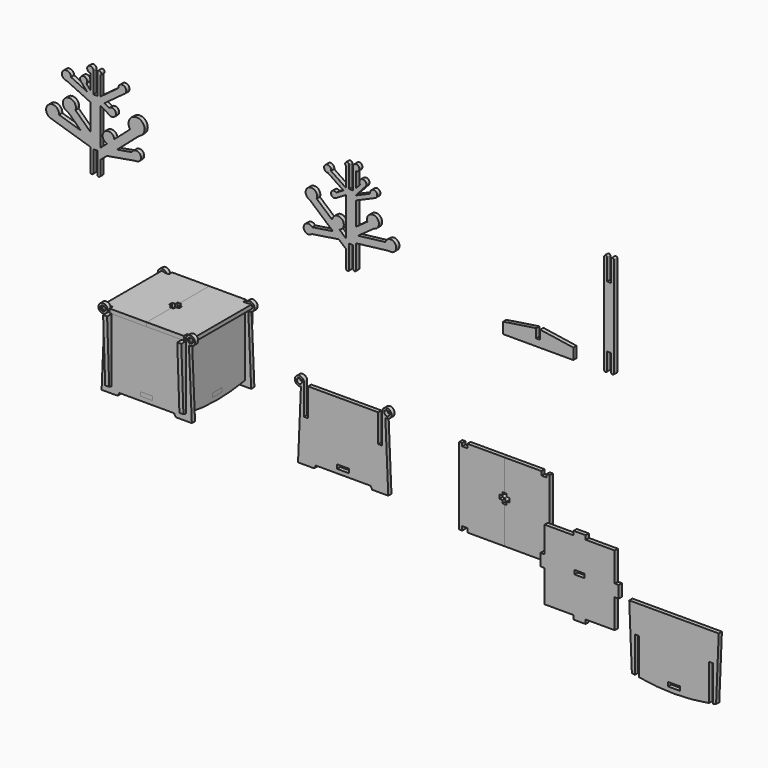
from build123d import *

# Parameters (mm, degrees)
F0_W      = 20
F0_H      = 60
F0_W_2    = 60
F0_H_2    = 20
F1_DEPTH  = 20
F2_W      = 145
F2_H      = 20
F3_DEPTH  = 20
F6_W      = 20
F6_H      = 140
F7_DEPTH  = 20
F9_W      = 15
F9_H      = 20
F9_H_2    = 15
F9_W_2    = 175
F9_W_3    = 185
F9_W_4    = 10
F10_DEPTH = 20
F13_DEPTH = 20
F18_DEPTH = 20
F19_W     = 15
F19_H     = 20
F19_W_2   = 20
F20_DEPTH = 335
F19_H_2   = 15
F21_DEPTH = 335
F23_ANGLE = 90
F27_ANGLE = -90


# Not quite as in the source:
# - a feature names something its author has since deleted; it is built from what else it names


with BuildPart() as f1:
    # F0 (on Top) → F1 (new body)
    with BuildSketch(Plane.XY):
        Polygon((394.9682962894, 292.9871472716), (249.9682962894, 292.9871472716), (249.9682962894, 133.2951399684), (269.9682962894, 133.2951399684), (269.9682962894, 73.2951399684), (249.9682962894, 73.2951399684), (249.9682962894, -57.0128527284), (394.9682962894, -57.0128527284), (394.9682962894, -37.0128527284), (454.9682962894, -37.0128527284), (454.9682962894, -57.0128527284), (599.9682962894, -57.0128527284), (599.9682962894, 87.9871472716), (579.9682962894, 87.9871472716), (579.9682962894, 147.9871472716), (599.9682962894, 147.9871472716), (599.9682962894, 292.9871472716), (454.9682962894, 292.9871472716), (454.9682962894, 272.9871472716), (394.9682962894, 272.9871472716), align=None)
        with Locations((239.9682962894, 103.2951399684)):
            Rectangle(F0_W, F0_H)
        with Locations((424.9682962894, 302.9871472716)):
            Rectangle(F0_W_2, F0_H_2)
        with Locations((609.9682962894, 117.9871472716)):
            Rectangle(F0_W, F0_H)
        with Locations((424.9682962894, -67.0128527284)):
            Rectangle(F0_W_2, F0_H_2)
        with Locations((424.9682962894, -47.0128527284)):
            Rectangle(F0_W_2, F0_H_2)
        with Locations((589.9682962894, 117.9871472716)):
            Rectangle(F0_W, F0_H)
        with Locations((424.9682962894, 282.9871472716)):
            Rectangle(F0_W_2, F0_H_2)
        with Locations((259.9682962894, 103.2951399684)):
            Rectangle(F0_W, F0_H)
    extrude(amount=F1_DEPTH)


with BuildPart() as f3:
    # F2 (on face) → F3 (new body)
    with BuildSketch(Plane.XZ.offset(57.0128527284)):
        Polygon((249.9682962894, 0), (249.9682962894, -35), (279.9682962894, -35), (288.6285503273, -20), (561.3080422516, -20), (569.9682962894, -35), (599.9682962894, -35), (599.9682962894, 175), (599.9682962894, 315), (249.9682962894, 315), (249.9682962894, 175), (249.9682962894, 20), (394.9682962894, 20), (394.9682962894, 0), align=None)
        with BuildLine():
            Line((199.9682962894, -35), (249.9682962894, -35))
            Line((249.9682962894, -35), (249.9682962894, 0))
            Line((249.9682962894, 0), (249.9682962894, 20))
            Line((249.9682962894, 20), (249.9682962894, 175))
            Line((249.9682962894, 175), (229.9682962894, 175))
            Line((229.9682962894, 175), (229.9682962894, 315))
            Line((229.9682962894, 315), (227.6933161634, 315))
            ThreePointArc((227.6933161634, 315), (222.2567695839, 307.7904363638), (214.4638373042, 303.2292903433))
            Line((214.4638373042, 303.2292903433), (199.9682962894, -35))
        make_face()
        with Locations((322.4682962894, 10)):
            Rectangle(F2_W, F2_H)
        with BuildLine():
            ThreePointArc((229.9682962894, 324.9736428261), (188.2413445442, 338.3265929994), (214.4638373042, 303.2292903433))
            Line((214.4638373042, 303.2292903433), (214.9561781187, 314.7172426837))
            ThreePointArc((214.9561781187, 314.7172426837), (195.2883462942, 330.681424191), (219.9682962894, 324.9736428261))
            ThreePointArc((219.9682962894, 324.9736428261), (218.7453349206, 319.4689756173), (215.3065484311, 315))
            Line((215.3065484311, 315), (227.6933161634, 315))
            ThreePointArc((227.6933161634, 315), (229.3923398265, 319.8587360382), (229.9682962894, 324.9736428261))
        make_face()
        with BuildLine():
            Line((214.9561781187, 314.7172426837), (214.4638373042, 303.2292903433))
            ThreePointArc((214.4638373042, 303.2292903433), (222.2567695839, 307.7904363638), (227.6933161634, 315))
            Line((227.6933161634, 315), (215.3065484311, 315))
            ThreePointArc((215.3065484311, 315), (215.1325874733, 314.8571044129), (214.9561781187, 314.7172426837))
        make_face()
        with BuildLine():
            Line((599.9682962894, 175), (599.9682962894, -35))
            Line((599.9682962894, -35), (649.9682962894, -35))
            Line((649.9682962894, -35), (635.4727552747, 303.2292903433))
            ThreePointArc((635.4727552747, 303.2292903433), (627.679822995, 307.7904363638), (622.2432764154, 315))
            Line((622.2432764154, 315), (619.9682962894, 315))
            Line((619.9682962894, 315), (619.9682962894, 175))
            Line((619.9682962894, 175), (599.9682962894, 175))
        make_face()
        with BuildLine():
            Line((229.9682962894, 315), (229.9682962894, 324.9736428261))
            ThreePointArc((229.9682962894, 324.9736428261), (229.3923398265, 319.8587360382), (227.6933161634, 315))
            Line((227.6933161634, 315), (229.9682962894, 315))
        make_face()
        with BuildLine():
            ThreePointArc((622.2432764154, 315), (627.679822995, 307.7904363638), (635.4727552747, 303.2292903433))
            Line((635.4727552747, 303.2292903433), (634.9804144601, 314.7172426837))
            ThreePointArc((634.9804144601, 314.7172426837), (634.8040051056, 314.8571044129), (634.6300441478, 315))
            Line((634.6300441478, 315), (627.7177929878, 315))
            Line((627.7177929878, 315), (622.2432764154, 315))
        make_face()
        with BuildLine():
            Line((634.9804144601, 314.7172426837), (635.4727552747, 303.2292903433))
            ThreePointArc((635.4727552747, 303.2292903433), (656.3212464628, 306.2466910808), (665.9682962894, 324.9736428261))
            ThreePointArc((665.9682962894, 324.9736428261), (642.9682962894, 347.9736428261), (619.9682962894, 324.9736428261))
            Line((619.9682962894, 324.9736428261), (627.7177929878, 324.9736428261))
            Line((627.7177929878, 324.9736428261), (627.7177929878, 315))
            Line((627.7177929878, 315), (634.6300441478, 315))
            ThreePointArc((634.6300441478, 315), (637.4636290807, 336.7506814573), (655.9682962894, 324.9736428261))
            ThreePointArc((655.9682962894, 324.9736428261), (648.6760776543, 313.2936928309), (634.9804144601, 314.7172426837))
        make_face()
        with BuildLine():
            Line((619.9682962894, 324.9736428261), (619.9682962894, 315))
            Line((619.9682962894, 315), (622.2432764154, 315))
            ThreePointArc((622.2432764154, 315), (620.5442527524, 319.8587360382), (619.9682962894, 324.9736428261))
        make_face()
        with BuildLine():
            ThreePointArc((619.9682962894, 324.9736428261), (620.5442527524, 319.8587360382), (622.2432764154, 315))
            Line((622.2432764154, 315), (627.7177929878, 315))
            Line((627.7177929878, 315), (627.7177929878, 324.9736428261))
            Line((627.7177929878, 324.9736428261), (619.9682962894, 324.9736428261))
        make_face()
    extrude(amount=F3_DEPTH)


with BuildPart() as f5_1:
    # F5: instance of F3
    add(f3.part.mirror(Plane(origin=(424.9682962894, 117.9871472716, 141.3924873425), x_dir=(1, 0, 0), z_dir=(0, 1, 0))))

    # F15: cut F1
    add(f1.part, mode=Mode.SUBTRACT)


with BuildPart() as f7:
    # F6 (on face) → F7 (new body)
    with BuildSketch(Plane.YZ.offset(599.9682962894)):
        with Locations((-67.0128527284, 245)):
            Rectangle(F6_W, F6_H)
        with BuildLine():
            Line((-77.0128527284, 315), (-105.1934603447, 315))
            Line((-105.1934603447, 315), (-92.0128527284, 0.2758802016))
            ThreePointArc((-92.0128527284, 0.2758802016), (117.9871472716, -22.1976265311), (327.9871472716, 0.2758802016))
            Line((327.9871472716, 0.2758802016), (341.167754888, 315))
            Line((341.167754888, 315), (-57.0128527284, 315))
            Line((-57.0128527284, 315), (-57.0128527284, 175))
            Line((-57.0128527284, 175), (-77.0128527284, 175))
            Line((-77.0128527284, 175), (-77.0128527284, 315))
        make_face()
    extrude(amount=F7_DEPTH)

    # F12 (on face) → F13 (cut, through all)
    with BuildSketch(Plane.YZ.offset(619.9682962894)):
        with BuildLine():
            Line((-57.0128527284, 175), (-77.0128527284, 175))
            Line((-77.0128527284, 175), (-77.0128527284, -2.8507864877))
            ThreePointArc((-77.0128527284, -2.8507864877), (-67.0225840557, -4.7996175192), (-57.0128527283, -6.645881123))
            Line((-57.0128527284, -6.645881123), (-57.0128527284, 175))
        make_face()
        with BuildLine():
            Line((292.9871472716, 175), (292.9871472716, -6.645881123))
            ThreePointArc((292.9871472716, -6.645881123), (302.996878599, -4.7996175192), (312.9871472716, -2.8507864877))
            Line((312.9871472716, -2.8507864877), (312.9871472716, 175))
            Line((312.9871472716, 175), (292.9871472716, 175))
        make_face()
    extrude(amount=-F13_DEPTH, mode=Mode.SUBTRACT)


with BuildPart() as f10:
    # F9 (on face) → F10 (new body)
    with BuildSketch(Plane.XY.offset(315)):
        Polygon((214.6351480484, 292.9871472716), (199.6351480484, 292.9871472716), (199.6351480484, -57.0128527284), (214.6351480484, -57.0128527284), (239.9682962894, -57.0128527284), (424.9682962894, -57.0128527284), (424.9682962894, 292.9871472716), (249.9682962894, 292.9871472716), (239.9682962894, 292.9871472716), align=None)
        with Locations((207.1351480484, 302.9871472716)):
            Rectangle(F9_W, F9_H)
        with Locations((207.1351480484, -64.5128527284)):
            Rectangle(F9_W, F9_H_2)
        with Locations((337.4682962894, 302.9871472716)):
            Rectangle(F9_W_2, F9_H)
        with Locations((332.4682962894, -67.0128527284)):
            Rectangle(F9_W_3, F9_H)
        with Locations((244.9682962894, 302.9871472716)):
            Rectangle(F9_W_4, F9_H)
    extrude(amount=F10_DEPTH)


with BuildPart() as f11_1:
    # F11: instance of F10
    add(f10.part.mirror(Plane(origin=(424.9682962894, 8.14114362, 10), x_dir=(0, -1, 0), z_dir=(-1, 0, 0))))


with BuildPart() as f14_1:
    # F14: instance of F7
    add(f7.part.mirror(Plane(origin=(424.9682962894, 8.14114362, 10), x_dir=(0, -1, 0), z_dir=(-1, 0, 0))))

    # F15: cut F1
    add(f1.part, mode=Mode.SUBTRACT)


with BuildPart() as f3_1:
    add(f3.part)

    # F15: cut F1
    add(f1.part, mode=Mode.SUBTRACT)


with BuildPart() as f7_1:
    add(f7.part)

    # F15: cut F1
    add(f1.part, mode=Mode.SUBTRACT)


with BuildPart() as f18:
    # F17 (on Front) → F18 (new body)
    with BuildSketch(Plane.XZ):
        with BuildLine():
            Line((1358.0063962936, 927.3299227427), (1358.0063962936, 852.0097017288))
            Line((1358.0063962936, 852.0097017288), (1373.0063962936, 852.0097017288))
            Line((1373.0063962936, 852.0097017288), (1373.0063962936, 957.0097017288))
            Line((1373.0063962936, 957.0097017288), (1383.0063962936, 957.0097017288))
            Line((1383.0063962936, 957.0097017288), (1393.0063962936, 957.0097017288))
            Line((1393.0063962936, 957.0097017288), (1393.0063962936, 852.0097017288))
            Line((1393.0063962936, 852.0097017288), (1408.0063962936, 852.0097017288))
            Line((1408.0063962936, 852.0097017288), (1408.0063962936, 969.9942015563))
            Line((1408.0063962936, 969.9942015563), (1408.0063962936, 999.8148856006))
            Line((1408.0063962936, 999.8148856006), (1408.0063962936, 1042.8129530404))
            Line((1408.0063962936, 1042.8129530404), (1408.0063962936, 1158.2306663639))
            Line((1408.0063962936, 1158.2306663639), (1408.0063962936, 1180.0459125289))
            Line((1408.0063962936, 1180.0459125289), (1408.0063962936, 1182.063221294))
            Line((1408.0063962936, 1182.063221294), (1408.0063962936, 1211.9989233637))
            Line((1408.0063962936, 1211.9989233637), (1408.0063962936, 1286.5059554373))
            ThreePointArc((1408.0063962936, 1286.5059554373), (1398.5303222166, 1289.7389980343), (1393.0063962936, 1298.0897337351))
            Line((1393.0063962936, 1298.0897337351), (1393.0063962936, 1197.0097017288))
            Line((1393.0063962936, 1197.0097017288), (1383.0063962936, 1197.0097017288))
            Line((1383.0063962936, 1197.0097017288), (1373.0063962936, 1197.0097017288))
            Line((1373.0063962936, 1197.0097017288), (1373.0063962936, 1300.6884193425))
            ThreePointArc((1373.0063962936, 1300.6884193425), (1367.8351965444, 1292.3296392908), (1358.0063962936, 1292.257553019))
            Line((1358.0063962936, 1292.257553019), (1358.0063962936, 1196.3302201938))
            Line((1358.0063962936, 1196.3302201938), (1358.0063962936, 1166.3210256539))
            Line((1358.0063962936, 1166.3210256539), (1358.0063962936, 973.7387951534))
            Line((1358.0063962936, 973.7387951534), (1358.0063962936, 927.3299227427))
        make_face()
        with BuildLine():
            Line((1307.0047526675, 1135.4528445172), (1358.0063962936, 1166.3210256539))
            Line((1358.0063962936, 1166.3210256539), (1358.0063962936, 1196.3302201938))
            Line((1358.0063962936, 1196.3302201938), (1282.3904902943, 1246.8759732111))
            ThreePointArc((1282.3904902943, 1246.8759732111), (1276.5746307703, 1237.5575284857), (1266.3509514986, 1233.5408113865))
            Line((1266.3509514986, 1233.5408113865), (1344.325273473, 1181.4185658335))
            Line((1344.325273473, 1181.4185658335), (1309.5296382124, 1160.3588921519))
            ThreePointArc((1309.5296382124, 1160.3588921519), (1282.5132309658, 1150.5167126394), (1307.0047526675, 1135.4528445172))
        make_face()
        with BuildLine():
            ThreePointArc((1266.3509514986, 1233.5408113865), (1276.5746307703, 1237.5575284857), (1282.3904902943, 1246.8759732111))
            ThreePointArc((1282.3904902943, 1246.8759732111), (1282.762294408, 1248.9302740178), (1282.8868198395, 1251.0142326355))
            ThreePointArc((1282.8868198395, 1251.0142326355), (1252.6761490461, 1263.0429003914), (1266.3509514986, 1233.5408113865))
        make_face()
        with BuildLine():
            ThreePointArc((1373.0063962936, 1301.6901874538), (1357.4453211978, 1309.7927838997), (1358.0063962936, 1292.257553019))
            ThreePointArc((1358.0063962936, 1292.257553019), (1367.8351965444, 1292.3296392908), (1373.0063962936, 1300.6884193425))
            Line((1373.0063962936, 1300.6884193425), (1373.0063962936, 1301.6901874538))
        make_face()
        with BuildLine():
            Line((1393.0063962936, 1302.0097017288), (1393.0063962936, 1298.0897337351))
            ThreePointArc((1393.0063962936, 1298.0897337351), (1398.5303222166, 1289.7389980343), (1408.0063962936, 1286.5059554373))
            ThreePointArc((1408.0063962936, 1286.5059554373), (1418.9692004302, 1291.0468975923), (1423.5101425852, 1302.0097017288))
            ThreePointArc((1423.5101425852, 1302.0097017288), (1409.9824978471, 1317.38699576), (1393.0063962936, 1305.9296697225))
            Line((1393.0063962936, 1305.9296697225), (1393.0063962936, 1302.0097017288))
        make_face()
        with BuildLine():
            ThreePointArc((1427.3128137465, 1233.5008094695), (1438.0714579444, 1226.9519090886), (1450.4412384602, 1229.3236281204))
            ThreePointArc((1450.4412384602, 1229.3236281204), (1456.4835850457, 1235.681838003), (1458.6817789078, 1244.1732883453))
            ThreePointArc((1458.6817789078, 1244.1732883453), (1435.5451527148, 1260.7406793639), (1427.3128137465, 1233.5008094695))
        make_face()
        with BuildLine():
            Line((1408.0063962936, 1211.9989233637), (1408.0063962936, 1182.063221294))
            Line((1408.0063962936, 1182.063221294), (1450.4412384602, 1229.3236281204))
            ThreePointArc((1450.4412384602, 1229.3236281204), (1438.0714579444, 1226.9519090886), (1427.3128137465, 1233.5008094695))
            Line((1427.3128137465, 1233.5008094695), (1408.0063962936, 1211.9989233637))
        make_face()
        with BuildLine():
            Line((1408.0063962936, 1180.0459125289), (1408.0063962936, 1158.2306663639))
            Line((1408.0063962936, 1158.2306663639), (1499.7094965653, 1198.17812131))
            ThreePointArc((1499.7094965653, 1198.17812131), (1486.4551423715, 1200.0284786999), (1478.3840142688, 1210.7036189199))
            Line((1478.3840142688, 1210.7036189199), (1408.0063962936, 1180.0459125289))
        make_face()
        with BuildLine():
            ThreePointArc((1478.3840142688, 1210.7036189199), (1486.4551423715, 1200.0284786999), (1499.7094965653, 1198.17812131))
            ThreePointArc((1499.7094965653, 1198.17812131), (1509.1582181707, 1204.4083664417), (1512.8180551529, 1215.1181697845))
            ThreePointArc((1512.8180551529, 1215.1181697845), (1493.0927142207, 1232.4761033521), (1478.3840142688, 1210.7036189199))
        make_face()
        with BuildLine():
            ThreePointArc((1521.6589260101, 1092.436671257), (1486.5391984138, 1121.9965831199), (1463.4063667209, 1082.347424823))
            ThreePointArc((1463.4063667209, 1082.347424823), (1476.3122319583, 1066.659181432), (1496.2551078461, 1062.790843346))
            ThreePointArc((1496.2551078461, 1062.790843346), (1514.4392404842, 1072.9159829377), (1521.6589260101, 1092.436671257))
        make_face()
        with BuildLine():
            Line((1408.0063962936, 1042.8129530404), (1408.0063962936, 999.8148856006))
            Line((1408.0063962936, 999.8148856006), (1417.1330068338, 1006.3278083349))
            Line((1417.1330068338, 1006.3278083349), (1496.2551078461, 1062.790843346))
            ThreePointArc((1496.2551078461, 1062.790843346), (1476.3122319583, 1066.659181432), (1463.4063667209, 1082.347424823))
            Line((1463.4063667209, 1082.347424823), (1408.0063962936, 1042.8129530404))
        make_face()
        with BuildLine():
            Line((1408.0063962936, 999.8148856006), (1408.0063962936, 969.9942015563))
            Line((1408.0063962936, 969.9942015563), (1571.3598927739, 989.4405810887))
            ThreePointArc((1571.3598927739, 989.4405810887), (1555.9848998202, 1002.5256891792), (1553.6892929599, 1022.5841201052))
            Line((1553.6892929599, 1022.5841201052), (1417.1330068338, 1006.3278083349))
            Line((1417.1330068338, 1006.3278083349), (1408.0063962936, 999.8148856006))
        make_face()
        with BuildLine():
            ThreePointArc((1553.6892929599, 1022.5841201052), (1555.9848998202, 1002.5256891792), (1571.3598927739, 989.4405810887))
            ThreePointArc((1571.3598927739, 989.4405810887), (1596.2472451249, 993.0942193096), (1607.7514156575, 1015.4634714127))
            ThreePointArc((1607.7514156575, 1015.4634714127), (1583.8424897181, 1042.7279939115), (1553.6892929599, 1022.5841201052))
        make_face()
        with BuildLine():
            Line((1288.1377893227, 1034.5762828528), (1324.2487674008, 1003.132959737))
            ThreePointArc((1324.2487674008, 1003.132959737), (1340.1288531164, 1013.485145171), (1346.2899994895, 1031.4123630524))
            ThreePointArc((1346.2899994895, 1031.4123630524), (1318.7121234446, 1060.531471623), (1288.1377893227, 1034.5762828528))
        make_face()
        with BuildLine():
            Line((1321.5282960597, 959.0929143135), (1358.0063962936, 927.3299227427))
            Line((1358.0063962936, 927.3299227427), (1358.0063962936, 973.7387951534))
            Line((1358.0063962936, 973.7387951534), (1324.2487674008, 1003.132959737))
            ThreePointArc((1324.2487674008, 1003.132959737), (1297.9774993747, 1009.4192377064), (1288.1377893227, 1034.5762828528))
            Line((1288.1377893227, 1034.5762828528), (1211.2027185781, 1101.5668330154))
            ThreePointArc((1211.2027185781, 1101.5668330154), (1197.1534189214, 1086.783173215), (1176.8293775574, 1085.0882512201))
            Line((1176.8293775574, 1085.0882512201), (1291.8234953438, 984.9581136714))
            Line((1291.8234953438, 984.9581136714), (1321.5282960597, 959.0929143135))
        make_face()
        with BuildLine():
            ThreePointArc((1213.421498179, 1112.6229763031), (1167.536130825, 1135.5202707774), (1176.8293775574, 1085.0882512201))
            ThreePointArc((1176.8293775574, 1085.0882512201), (1197.1534189214, 1086.783173215), (1211.2027185781, 1101.5668330154))
            ThreePointArc((1211.2027185781, 1101.5668330154), (1212.8613280902, 1106.9846856199), (1213.421498179, 1112.6229763031))
        make_face()
        with BuildLine():
            ThreePointArc((1188.2260334932, 969.3581600213), (1146.1395737103, 956.7221845452), (1186.2245751985, 938.718556328))
            ThreePointArc((1186.2245751985, 938.718556328), (1191.2310014618, 946.2890948102), (1192.9875297533, 955.1936984062))
            ThreePointArc((1192.9875297533, 955.1936984062), (1191.7653026305, 962.6653752508), (1188.2260334932, 969.3581600213))
        make_face()
        with BuildLine():
            Line((1186.2245751985, 938.718556328), (1321.5282960597, 959.0929143135))
            Line((1321.5282960597, 959.0929143135), (1291.8234953438, 984.9581136714))
            Line((1291.8234953438, 984.9581136714), (1188.2260334932, 969.3581600213))
            ThreePointArc((1188.2260334932, 969.3581600213), (1191.7653026305, 962.6653752508), (1192.9875297533, 955.1936984062))
            ThreePointArc((1192.9875297533, 955.1936984062), (1191.2310014618, 946.2890948102), (1186.2245751985, 938.718556328))
        make_face()
        with BuildLine():
            ThreePointArc((1288.1377893227, 1034.5762828528), (1297.9774993747, 1009.4192377064), (1324.2487674008, 1003.132959737))
            Line((1324.2487674008, 1003.132959737), (1288.1377893227, 1034.5762828528))
        make_face()
        with BuildLine():
            Line((1373.0063962936, 852.0097017288), (1358.0063962936, 852.0097017288))
            Line((1358.0063962936, 852.0097017288), (1358.0063962936, 842.1414494514))
            ThreePointArc((1358.0063962936, 842.1414494514), (1365.5063962936, 834.6414494514), (1373.0063962936, 842.1414494514))
            Line((1373.0063962936, 842.1414494514), (1373.0063962936, 852.0097017288))
        make_face()
        with BuildLine():
            Line((1408.0063962936, 852.0097017288), (1393.0063962936, 852.0097017288))
            ThreePointArc((1393.0063962936, 852.0097017288), (1400.5063962936, 844.5097017288), (1408.0063962936, 852.0097017288))
        make_face()
    extrude(amount=-F18_DEPTH)


with BuildPart() as f18b:
    # F17 (on Front) → F18, piece 2 (new body)
    with BuildSketch(Plane.XZ):
        with BuildLine():
            Line((131.7743873596, 852.0097017288), (131.7743873596, 920.7000838269))
            Line((131.7743873596, 920.7000838269), (131.7743873596, 973.7387951534))
            Line((131.7743873596, 973.7387951534), (131.7743873596, 1160.476553513))
            Line((131.7743873596, 1160.476553513), (131.7743873596, 1198.8398938785))
            Line((131.7743873596, 1198.8398938785), (131.7743873596, 1292.257553019))
            ThreePointArc((131.7743873596, 1292.257553019), (121.9455871089, 1292.3296392908), (116.7743873596, 1300.6884193425))
            Line((116.7743873596, 1300.6884193425), (116.7743873596, 1197.0097017288))
            Line((116.7743873596, 1197.0097017288), (96.7743873596, 1197.0097017288))
            Line((96.7743873596, 1197.0097017288), (96.7743873596, 1298.0897337351))
            ThreePointArc((96.7743873596, 1298.0897337351), (91.2504614366, 1289.7389980343), (81.7743873596, 1286.5059554373))
            Line((81.7743873596, 1286.5059554373), (81.7743873596, 1211.9989233637))
            Line((81.7743873596, 1211.9989233637), (81.7743873596, 1191.795293997))
            Line((81.7743873596, 1191.795293997), (81.7743873596, 1181.3073472499))
            Line((81.7743873596, 1181.3073472499), (81.7743873596, 1158.63777396))
            Line((81.7743873596, 1158.63777396), (81.7743873596, 1028.6745173249))
            Line((81.7743873596, 1028.6745173249), (81.7743873596, 1004.0170956668))
            Line((81.7743873596, 1004.0170956668), (81.7743873596, 962.1281741858))
            Line((81.7743873596, 962.1281741858), (81.7743873596, 852.0097017288))
            ThreePointArc((81.7743873596, 852.0097017288), (89.2743873596, 844.5097017288), (96.7743873596, 852.0097017288))
            Line((96.7743873596, 852.0097017288), (96.7743873596, 957.0097017288))
            Line((96.7743873596, 957.0097017288), (116.7743873596, 957.0097017288))
            Line((116.7743873596, 957.0097017288), (116.7743873596, 852.0097017288))
            ThreePointArc((116.7743873596, 852.0097017288), (124.2743873596, 844.5097017288), (131.7743873596, 852.0097017288))
        make_face()
        with BuildLine():
            ThreePointArc((81.7743873596, 1286.5059554373), (91.2504614366, 1289.7389980343), (96.7743873596, 1298.0897337351))
            ThreePointArc((96.7743873596, 1298.0897337351), (97.1516813908, 1300.0336001754), (97.2781336511, 1302.0097017288))
            ThreePointArc((97.2781336511, 1302.0097017288), (70.8115832231, 1312.9725058653), (81.7743873596, 1286.5059554373))
        make_face()
        with BuildLine():
            ThreePointArc((116.7743873596, 1300.6884193425), (121.9455871089, 1292.3296392908), (131.7743873596, 1292.257553019))
            ThreePointArc((131.7743873596, 1292.257553019), (135.6594561935, 1295.9927867822), (137.0884230127, 1301.1893033981))
            ThreePointArc((137.0884230127, 1301.1893033981), (127.1757481731, 1311.3494083355), (116.7743873596, 1301.6901874538))
            Line((116.7743873596, 1301.6901874538), (116.7743873596, 1300.6884193425))
        make_face()
        with BuildLine():
            Line((131.7743873596, 1198.8398938785), (131.7743873596, 1160.476553513))
            Line((131.7743873596, 1160.476553513), (177.5853195244, 1132.7499931208))
            ThreePointArc((177.5853195244, 1132.7499931208), (209.7950897267, 1149.6529344664), (175.9433850891, 1162.9661164956))
            Line((175.9433850891, 1162.9661164956), (152.7273181512, 1177.0173844268))
            Line((152.7273181512, 1177.0173844268), (249.0520578394, 1248.0847968826))
            ThreePointArc((249.0520578394, 1248.0847968826), (230.9448813752, 1249.5189842242), (221.4657405593, 1265.0132613041))
            Line((221.4657405593, 1265.0132613041), (131.7743873596, 1198.8398938785))
        make_face()
        with BuildLine():
            ThreePointArc((261.4054288721, 1266.565301893), (240.6288228766, 1286.5502182833), (221.4657405593, 1265.0132613041))
            ThreePointArc((221.4657405593, 1265.0132613041), (230.9448813752, 1249.5189842242), (249.0520578394, 1248.0847968826))
            ThreePointArc((249.0520578394, 1248.0847968826), (258.0327043456, 1255.4507299117), (261.4054288721, 1266.565301893))
        make_face()
        with BuildLine():
            Line((164.4710962271, 949.1704614367), (215.3120596137, 993.4397923817))
            Line((215.3120596137, 993.4397923817), (325.5633307906, 1089.4401370981))
            ThreePointArc((325.5633307906, 1089.4401370981), (300.8157906129, 1089.0581578833), (280.5809961214, 1103.3108679714))
            Line((280.5809961214, 1103.3108679714), (201.6429943305, 1034.5762828528))
            ThreePointArc((201.6429943305, 1034.5762828528), (201.7720683942, 1032.9966626673), (201.8151354835, 1031.4123630524))
            ThreePointArc((201.8151354835, 1031.4123630524), (190.580177705, 1008.4113337656), (165.5320162525, 1003.132959737))
            Line((165.5320162525, 1003.132959737), (131.7743873596, 973.7387951534))
            Line((131.7743873596, 973.7387951534), (131.7743873596, 920.7000838269))
            Line((131.7743873596, 920.7000838269), (164.4710962271, 949.1704614367))
        make_face()
        with BuildLine():
            ThreePointArc((280.5809961214, 1103.3108679714), (300.8157906129, 1089.0581578833), (325.5633307906, 1089.4401370981))
            ThreePointArc((325.5633307906, 1089.4401370981), (345.1481220887, 1104.0273843311), (352.602519989, 1127.2821426392))
            ThreePointArc((352.602519989, 1127.2821426392), (299.9704369206, 1165.2351461745), (280.5809961214, 1103.3108679714))
        make_face()
        with BuildLine():
            Line((165.5320162525, 1003.132959737), (201.6429943305, 1034.5762828528))
            ThreePointArc((201.6429943305, 1034.5762828528), (153.5026353686, 1053.4054883984), (165.5320162525, 1003.132959737))
        make_face()
        with BuildLine():
            ThreePointArc((307.726123849, 973.8374211464), (290.8963475898, 985.7131378543), (289.9314294615, 1006.2884373483))
            Line((289.9314294615, 1006.2884373483), (215.3120596137, 993.4397923817))
            Line((215.3120596137, 993.4397923817), (164.4710962271, 949.1704614367))
            Line((164.4710962271, 949.1704614367), (307.726123849, 973.8374211464))
        make_face()
        with BuildLine():
            ThreePointArc((307.726123849, 973.8374211464), (326.6616617294, 979.1363861977), (334.9058313357, 996.9876408577))
            ThreePointArc((334.9058313357, 996.9876408577), (316.2057178488, 1019.9506635208), (289.9314294615, 1006.2884373483))
            ThreePointArc((289.9314294615, 1006.2884373483), (290.8963475898, 985.7131378543), (307.726123849, 973.8374211464))
        make_face()
        with BuildLine():
            ThreePointArc((201.8151354835, 1031.4123630524), (201.7720683942, 1032.9966626673), (201.6429943305, 1034.5762828528))
            Line((201.6429943305, 1034.5762828528), (165.5320162525, 1003.132959737))
            ThreePointArc((165.5320162525, 1003.132959737), (190.580177705, 1008.4113337656), (201.8151354835, 1031.4123630524))
        make_face()
        with BuildLine():
            Line((-115.3886328976, 1023.4316359259), (81.7743873596, 962.1281741858))
            Line((81.7743873596, 962.1281741858), (81.7743873596, 1004.0170956668))
            Line((81.7743873596, 1004.0170956668), (34.1432376901, 1018.8269436677))
            Line((34.1432376901, 1018.8269436677), (-73.6147060184, 1052.3318827313))
            ThreePointArc((-73.6147060184, 1052.3318827313), (-87.5478043451, 1027.8302793288), (-115.3886328976, 1023.4316359259))
        make_face()
        with BuildLine():
            Line((34.1432376901, 1018.8269436677), (81.7743873596, 1004.0170956668))
            Line((81.7743873596, 1004.0170956668), (81.7743873596, 1028.6745173249))
            Line((81.7743873596, 1028.6745173249), (8.1144947349, 1098.9279843716))
            ThreePointArc((8.1144947349, 1098.9279843716), (-6.436711384, 1082.0512289569), (-28.437850559, 1078.5139492333))
            Line((-28.437850559, 1078.5139492333), (34.1432376901, 1018.8269436677))
        make_face()
        with BuildLine():
            ThreePointArc((-28.437850559, 1078.5139492333), (-6.436711384, 1082.0512289569), (8.1144947349, 1098.9279843716))
            ThreePointArc((8.1144947349, 1098.9279843716), (9.6865730628, 1104.5816994493), (10.2163565159, 1110.4259490967))
            ThreePointArc((10.2163565159, 1110.4259490967), (-42.9746834539, 1135.4884881733), (-28.437850559, 1078.5139492333))
        make_face()
        with BuildLine():
            Line((-115.9862366891, 1023.6174475508), (-115.3886328976, 1023.4316359259))
            ThreePointArc((-115.3886328976, 1023.4316359259), (-87.5478043451, 1027.8302793288), (-73.6147060184, 1052.3318827313))
            ThreePointArc((-73.6147060184, 1052.3318827313), (-73.5574869741, 1053.4440685801), (-73.5384064913, 1054.5575618744))
            ThreePointArc((-73.5384064913, 1054.5575618744), (-125.1818847355, 1080.8211724547), (-115.9862366891, 1023.6174475508))
        make_face()
        with BuildLine():
            Line((-36.7222297475, 1214.4167181183), (81.7743873596, 1158.63777396))
            Line((81.7743873596, 1158.63777396), (81.7743873596, 1181.3073472499))
            Line((81.7743873596, 1181.3073472499), (65.8842164793, 1199.2751442733))
            Line((65.8842164793, 1199.2751442733), (-14.5381002884, 1237.1316841947))
            ThreePointArc((-14.5381002884, 1237.1316841947), (-14.5373142342, 1237.0231011095), (-14.5370522141, 1236.9145154953))
            ThreePointArc((-14.5370522141, 1236.9145154953), (-21.01622974, 1221.1163115705), (-36.7222297475, 1214.4167181183))
        make_face()
        with BuildLine():
            ThreePointArc((-14.5381002884, 1237.1316841947), (-53.1339306838, 1252.6352185181), (-36.7222297475, 1214.4167181183))
            ThreePointArc((-36.7222297475, 1214.4167181183), (-21.01622974, 1221.1163115705), (-14.5370522141, 1236.9145154953))
            ThreePointArc((-14.5370522141, 1236.9145154953), (-14.5373142342, 1237.0231011095), (-14.5381002884, 1237.1316841947))
        make_face()
        with BuildLine():
            Line((81.7743873596, 1191.795293997), (81.7743873596, 1211.9989233637))
            Line((81.7743873596, 1211.9989233637), (62.4679699068, 1233.5008094695))
            ThreePointArc((62.4679699068, 1233.5008094695), (51.6711699178, 1226.9450614733), (39.2738473938, 1229.3647961747))
            Line((39.2738473938, 1229.3647961747), (65.8842164793, 1199.2751442733))
            Line((65.8842164793, 1199.2751442733), (81.7743873596, 1191.795293997))
        make_face()
        with BuildLine():
            ThreePointArc((39.2738473938, 1229.3647961747), (51.6711699178, 1226.9450614733), (62.4679699068, 1233.5008094695))
            ThreePointArc((62.4679699068, 1233.5008094695), (65.166395764, 1238.5366621524), (66.0990047455, 1244.1732883453))
            ThreePointArc((66.0990047455, 1244.1732883453), (40.1414712296, 1259.4938668862), (39.2738473938, 1229.3647961747))
        make_face()
        Polygon((81.7743873596, 1181.3073472499), (81.7743873596, 1191.795293997), (65.8842164793, 1199.2751442733), align=None)
    extrude(amount=-F18_DEPTH)


with BuildPart() as f18c:
    # F17 (on Front) → F18, piece 3 (new body)
    with BuildSketch(Plane.XZ):
        Polygon((2140.8269119263, 809.2685198784), (2490.8269119263, 809.2685198784), (2490.8269119263, 864.2685198784), (2325.8269119263, 889.2685198784), (2325.8269119263, 844.2685198784), (2315.8269119263, 844.2685198784), (2305.8269119263, 844.2685198784), (2305.8269119263, 889.2685198784), (2140.8269119263, 864.2685198784), align=None)
    extrude(amount=-F18_DEPTH)


with BuildPart() as f18d:
    # F17 (on Front) → F18, piece 4 (new body)
    with BuildSketch(Plane.XZ):
        with BuildLine():
            ThreePointArc((2694.5608949661, 1314.2685198784), (2687.0608949661, 1321.7685198784), (2679.5608949661, 1314.2685198784))
            Line((2679.5608949661, 1314.2685198784), (2679.5608949661, 1209.2685198784))
            Line((2679.5608949661, 1209.2685198784), (2669.5608949661, 1209.2685198784))
            Line((2669.5608949661, 1209.2685198784), (2659.5608949661, 1209.2685198784))
            Line((2659.5608949661, 1209.2685198784), (2659.5608949661, 1314.2685198784))
            ThreePointArc((2659.5608949661, 1314.2685198784), (2652.0608949661, 1321.7685198784), (2644.5608949661, 1314.2685198784))
            Line((2644.5608949661, 1314.2685198784), (2644.5608949661, 816.7685198784))
            ThreePointArc((2644.5608949661, 816.7685198784), (2652.0608949661, 809.2685198784), (2659.5608949661, 816.7685198784))
            Line((2659.5608949661, 816.7685198784), (2659.5608949661, 901.7685198784))
            Line((2659.5608949661, 901.7685198784), (2679.5608949661, 901.7685198784))
            Line((2679.5608949661, 901.7685198784), (2679.5608949661, 816.7685198784))
            ThreePointArc((2679.5608949661, 816.7685198784), (2687.0608949661, 809.2685198784), (2694.5608949661, 816.7685198784))
            Line((2694.5608949661, 816.7685198784), (2694.5608949661, 1314.2685198784))
        make_face()
    extrude(amount=-F18_DEPTH)


with BuildPart() as f20_tool:
    # F19 (on face) → F20 (new body, through all)
    with BuildSketch(Plane(origin=(0, 0, 0), x_dir=(1, 0, 0), z_dir=(0, 0, -1))):
        with Locations((442.4682962894, -103.2951399684)):
            Rectangle(F19_W, F19_H)
        with Locations((407.4682962894, -103.2951399684)):
            Rectangle(F19_W, F19_H)
        with Locations((424.9682962894, -103.2951399684)):
            Rectangle(F19_W_2, F19_H)
    extrude(amount=-F20_DEPTH)


with BuildPart() as f1_1:
    add(f1.part)

    # F20: cut by f20_tool
    add(f20_tool.part, mode=Mode.SUBTRACT)


with BuildPart() as f10_1:
    add(f10.part)

    # F20: cut by f20_tool
    add(f20_tool.part, mode=Mode.SUBTRACT)


with BuildPart() as f11_1_1:
    add(f11_1.part)

    # F20: cut by f20_tool
    add(f20_tool.part, mode=Mode.SUBTRACT)


with BuildPart() as f21_tool:
    # F19 (on face) → F21 (new body, through all)
    with BuildSketch(Plane(origin=(0, 0, 0), x_dir=(1, 0, 0), z_dir=(0, 0, -1))):
        with Locations((424.9682962894, -120.7951399684)):
            Rectangle(F19_W_2, F19_H_2)
        with Locations((424.9682962894, -85.7951399684)):
            Rectangle(F19_W_2, F19_H_2)
        with Locations((424.9682962894, -103.2951399684)):
            Rectangle(F19_W_2, F19_H)
    extrude(amount=-F21_DEPTH)


with BuildPart() as f10_2:
    add(f10_1.part)

    # F21: cut by f21_tool
    add(f21_tool.part, mode=Mode.SUBTRACT)


with BuildPart() as f11_1_2:
    add(f11_1_1.part)

    # F21: cut by f21_tool
    add(f21_tool.part, mode=Mode.SUBTRACT)


with BuildPart() as f22_1:
    # F22: copy of F11_1
    add(f11_1_2.part.moved(Location((1800, 0, 0))))


with BuildPart() as f22_2:
    # F22: copy of F10
    add(f10_2.part.moved(Location((1800, 0, 0))))


with BuildPart() as f22_3:
    # F22: copy of F1
    add(f1_1.part.moved(Location((1800, 0, 0))))


with BuildPart() as f22_1_1:
    # F23: moved
    add(f22_1.part.rotate(Axis((2132.4682962894, -77.0128527284, 335), (-1, 0, 0)), F23_ANGLE))


with BuildPart() as f22_2_1:
    # F23: moved
    add(f22_2.part.rotate(Axis((2132.4682962894, -77.0128527284, 335), (-1, 0, 0)), F23_ANGLE))


with BuildPart() as f22_3_1:
    # F23: moved
    add(f22_3.part.rotate(Axis((2132.4682962894, -77.0128527284, 335), (-1, 0, 0)), F23_ANGLE))


with BuildPart() as f24_1:
    # F24: copy of F3
    add(f3_1.part.moved(Location((979.64182, 0, 0))))


with BuildPart() as f22_3_2:
    # F25: moved
    add(f22_3_1.part.moved(Location((626.97816, 0, 0))))


with BuildPart() as f26_1:
    # F26: copy of F7
    add(f7_1.part.moved(Location((2700, 0, 0))))


with BuildPart() as f26_1_1:
    # F27: moved
    add(f26_1.part.rotate(Axis((3026.9464562894, -412.0128527284, 37.5), (0, 0, 1)), F27_ANGLE))


solid = Compound([f5_1.part, f14_1.part, f3_1.part, f7_1.part, f18.part, f18b.part, f18c.part, f18d.part, f1_1.part, f10_2.part, f11_1_2.part, f22_1_1.part, f22_2_1.part, f24_1.part, f22_3_2.part, f26_1_1.part])
